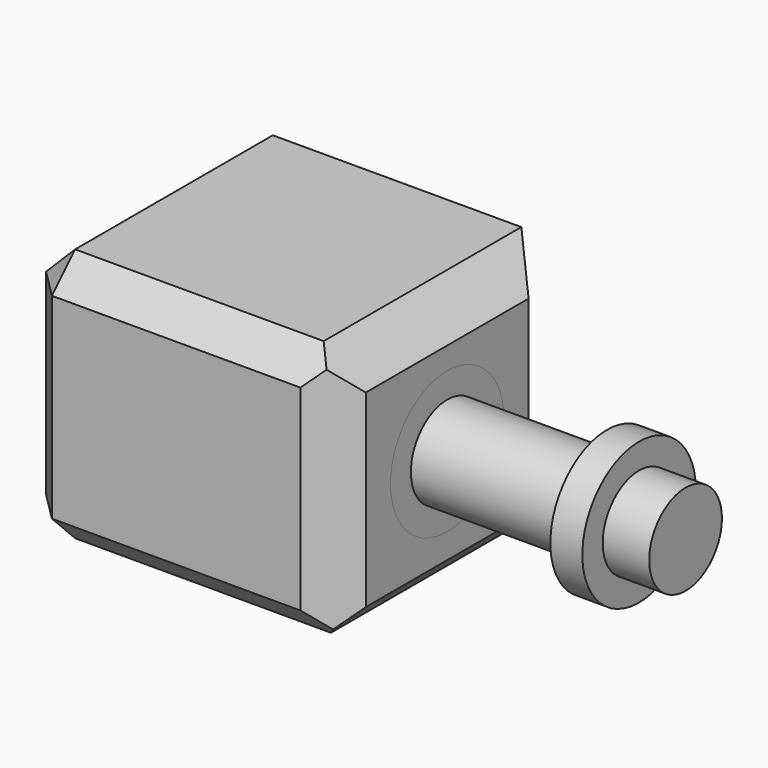
from build123d import *

# Parameters (mm, degrees)
F0_W     = 54.864
F0_H     = 48.26
F1_DEPTH = 44.45
F2_R     = 7.9426697317
F3_DEPTH = 41.656
F2_R_2   = 12.3876697317
F4_DEPTH = 33.528
F5_DEPTH = 36.83
F6_DEPTH = 27.94
F2_W     = 48.26
F2_H     = 44.45
F7_DEPTH = 54.864
F8_DEPTH = 54.864
F9_SIZE  = 6.35
F10_SIZE = 5.08


with BuildPart() as f1:
    # F0 (on Top) → F1 (new body)
    with BuildSketch(Plane.XY):
        with Locations((-94.6675501764, 11.3354255426)):
            Rectangle(F0_W, F0_H)
    extrude(amount=F1_DEPTH)

    # F5 (cut): a face of the model
    f5_faces = [f1.faces().sort_by_distance(p)[0] for p in [
        (-94.6675501764, 11.3354255426, 44.45),
    ]]
    extrude(f5_faces, amount=-F5_DEPTH, mode=Mode.SUBTRACT)

    # F2 (on face) → F7 (join, through all)
    with BuildSketch(Plane.YZ.offset(-67.2355501764)):
        with Locations((11.3354255426, 22.225)):
            Rectangle(F2_W, F2_H)
        with Locations((11.3357125817, 21.8364697298)):
            Circle(F2_R_2, mode=Mode.SUBTRACT)
    extrude(amount=-F7_DEPTH)

    # F9
    f9_edges = [f1.edges().sort_by_distance(p)[0] for p in [
        (-67.23555, 11.335426, 44.45),
        (-67.23555, -12.794574, 22.225),
        (-67.23555, 35.465426, 22.225),
    ]]
    chamfer(f9_edges, length=F9_SIZE)

    # F10 (call 1 of 2: OpenCascade refuses the feature's edges together)
    f10_edges = [f1.edges().sort_by_distance(p)[0] for p in [
        (-97.84255, -12.794574, 0),
        (-122.09955, -12.794574, 22.225),
        (-122.09955, 11.335426, 44.45),
        (-122.09955, 35.465426, 22.225),
        (-97.84255, 35.465426, 0),
        (-122.09955, 11.335426, 0),
        (-97.84255, -12.794574, 44.45),
    ]]
    chamfer(f10_edges, length=F10_SIZE)

    # F10#2 (call 2 of 2)
    f10_2_edges = [f1.edges().sort_by_distance(p)[0] for p in [
        (-67.23555, 11.335426, 0),
    ]]
    chamfer(f10_2_edges, length=F10_SIZE)


with BuildPart() as f3:
    # F2 (on face) → F3 (new body)
    with BuildSketch(Plane.YZ.offset(-67.2355501764)):
        with Locations((11.3357125817, 21.8364697298)):
            Circle(F2_R)
    extrude(amount=F3_DEPTH)

    # F2 (on face) → F4 (join)
    with BuildSketch(Plane.YZ.offset(-67.2355501764)):
        with Locations((11.3357125817, 21.8364697298)):
            Circle(F2_R_2)
        with Locations((11.3357125817, 21.8364697298)):
            Circle(F2_R, mode=Mode.SUBTRACT)
    extrude(amount=F4_DEPTH)

    # F2 (on face) → F6 (cut)
    with BuildSketch(Plane.YZ.offset(-67.2355501764)):
        with Locations((11.3357125817, 21.8364697298)):
            Circle(F2_R_2)
        with Locations((11.3357125817, 21.8364697298)):
            Circle(F2_R, mode=Mode.SUBTRACT)
    extrude(amount=F6_DEPTH, mode=Mode.SUBTRACT)

    # F2 (on face) → F8 (join, through all)
    with BuildSketch(Plane.YZ.offset(-67.2355501764)):
        with Locations((11.3357125817, 21.8364697298)):
            Circle(F2_R_2)
        with Locations((11.3357125817, 21.8364697298)):
            Circle(F2_R, mode=Mode.SUBTRACT)
        with Locations((11.3357125817, 21.8364697298)):
            Circle(F2_R)
    extrude(amount=-F8_DEPTH)


solid = Compound([f1.part, f3.part])
